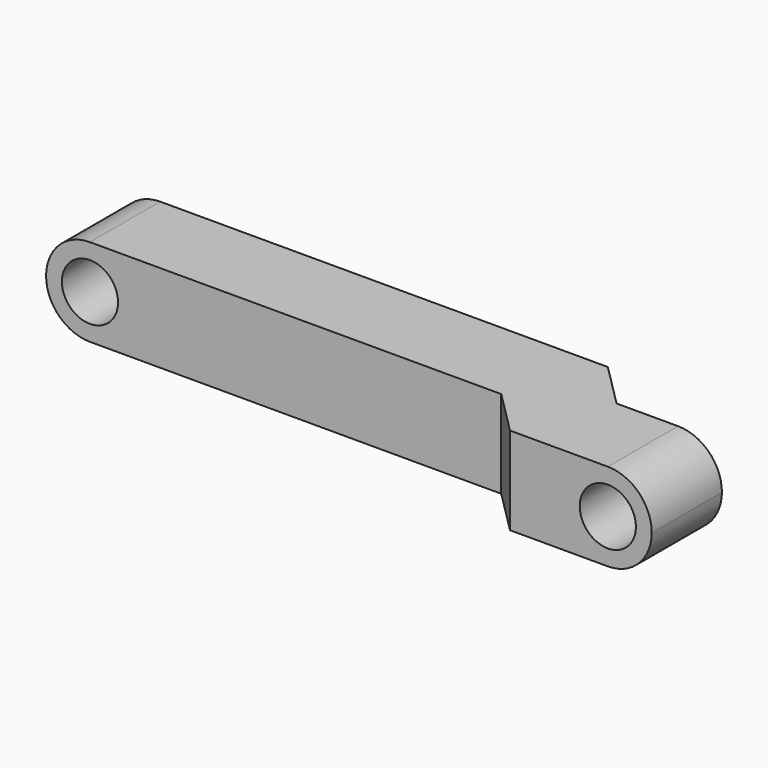
from build123d import *

# Parameters (mm, degrees)
F1_DEPTH = 7.9375
F2_R     = 3.96874
F3_R     = 2.54
F4_DEPTH = 11.90625


# Not quite as in the source:
# - a fillet or chamfer is up to 0.001 mm smaller than in the source, because OpenCascade refuses the exact size


with BuildPart() as f1:
    # F0 (on Top) → F1 (new body)
    with BuildSketch(Plane.XY):
        Polygon((44.45, 0), (0, 0), (0, -7.9375), (41.1621798487, -7.9375), (45.1309298487, -11.90625), (57.94375, -11.90625), (57.94375, -3.96875), (48.41875, -3.96875), align=None)
    extrude(amount=F1_DEPTH)

    # F2 (radius 3.96875 in the source; OpenCascade refuses exactly that, so slightly less here)
    f2_edges = [f1.edges().sort_by_distance(p)[0] for p in [
        (0, -3.96875, 0),
        (0, -3.96875, 7.9375),
        (57.94375, -7.9375, 0),
        (57.94375, -7.9375, 7.9375),
    ]]
    fillet(f2_edges, radius=F2_R)

    # F3 (on face) → F4 (cut, through all)
    with BuildSketch(Plane(origin=(0, 0, 0), x_dir=(-1, 0, 0), z_dir=(0, 1, 0))):
        with Locations((-3.96875, 3.96875)):
            Circle(F3_R)
        with Locations((-53.975, 3.96875)):
            Circle(F3_R)
    extrude(amount=-F4_DEPTH, mode=Mode.SUBTRACT)


solid = f1.part
